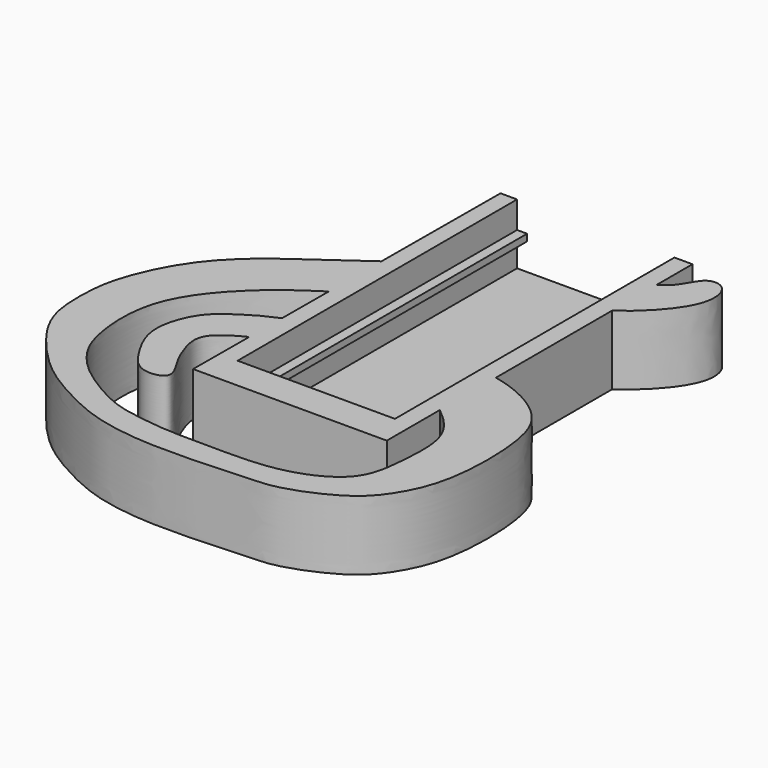
from build123d import *

# Parameters (mm, degrees)
F1_DEPTH = 50.8
F3_DEPTH = 50.8
F5_DEPTH = 44.45
F6_W     = 254.6858
F6_H     = 5
F8_DEPTH = 7.35
F7_W     = 254.6858
F7_H     = 5
F9_DEPTH = 7.35


# Not quite as in the source:
# - a feature names something its author has since deleted; it is built from what else it names


with BuildPart() as f1:
    # F0 (on Top) → F1 (new body)
    with BuildSketch(Plane.XY):
        with BuildLine():
            add(Edge.make_bspline(
                [(125.7269519745, 189.991159727), (122.3518203117, 192.7053935071), (111.2142106452, 193.3446218107), (104.5456392327, 168.8066823722), (63.3828372069, 157.6227686534), (21.7593119292, 134.7341899142), (0.3729918982, 123.8433966761), (-15.1527288368, 114.8249276639), (-32.5222819083, 102.4849064348), (-46.5725102285, 93.0684693464), (-82.8428413228, 66.746362756), (-103.7020746054, 52.59908065), (-127.8336751098, 28.9686859932), (-143.8102254505, 0.8754533738), (-152.6634719103, -25.1509877278), (-154.2263316972, -47.3151282142), (-153.2484361466, -77.7567714177), (-132.8958418183, -107.014281773), (-110.0491810359, -130.0752708141), (-88.0866600926, -143.6400857549), (-65.2385297743, -155.4769333183), (-41.5922440709, -163.1681919134), (-13.914670611, -166.3977513748), (0.1085926371, -166.5083652123), (26.8392485047, -166.7358495621), (61.2852961489, -163.9575559504), (81.9521897052, -164.4287242821), (122.6582829084, -147.5772914557), (140.1978462225, -126.7206556597), (155.9101153518, -94.4380334629), (156.0404662598, -30.3602794916), (141.7132105707, 3.4864205982), (88.6639491361, 30.0686559843), (11.8132162579, 20.380503993), (-18.3618763566, 13.3301979311), (-52.7384990739, 0.8286088804), (-69.2888621609, -9.4499896277), (-87.814391491, -22.1003193455), (-98.9611253924, -54.5390594087), (-85.3226254433, -80.4238827983), (-71.52170574, -100.1793594961), (-48.2690443764, -95.8332432139), (-57.7527638639, -80.2341547689), (-63.2820519632, -70.5245811939), (-69.3292706473, -54.6476744178), (-69.0979393699, -34.4305695104), (-2.6770546021, -7.9969048242), (42.314195006, -8.4277855233), (76.7904027335, -14.8362639415), (113.623336984, -42.8145575479), (119.3071426582, -68.2251948608), (117.588169986, -93.865138267), (114.1021059505, -125.7508497194), (80.0928160091, -144.2145120801), (45.4099166878, -147.7864485576), (16.1264360325, -146.9423859654), (-10.9926329062, -147.4579010438), (-39.004843071, -143.6649208598), (-58.6128504466, -139.0958568827), (-90.6420113734, -120.0345858112), (-105.7635321902, -103.2078654179), (-116.8591559372, -83.8529779262), (-122.0692191616, -29.7766902474), (-92.1392604492, 10.0671541536), (-65.3654050247, 33.2195527597), (-36.9417942364, 50.8675460638), (-7.1128182808, 72.0646516488), (12.800500031, 81.5981832557), (52.6243890024, 106.9180592515), (96.2625139742, 123.5069711027), (135.4755268537, 165.3473328003), (130.2770433606, 186.3320397352), (125.7269519745, 189.991159727)],
                knots=[0, 0, 0, 0, 0.0088413891, 0.0206204161, 0.0373502029, 0.0555383956, 0.0681302702, 0.0790631849, 0.090740175, 0.1017476271, 0.1188978604, 0.1323874644, 0.1471930925, 0.1620886022, 0.1755330322, 0.1877160253, 0.2017701538, 0.2171938111, 0.2320126089, 0.2451600157, 0.2582005547, 0.2713707729, 0.2848604147, 0.2945916029, 0.3079670972, 0.3231873767, 0.3352683463, 0.3520480663, 0.3655015892, 0.3808848218, 0.4014536445, 0.4167270326, 0.4360395597, 0.4587108082, 0.4735990292, 0.4888841325, 0.5003891776, 0.5123929862, 0.5269460027, 0.5408862436, 0.5532959287, 0.5634763718, 0.5728623362, 0.582057186, 0.5924855666, 0.602819313, 0.6239517883, 0.64185999, 0.6570853261, 0.6742212093, 0.687072608, 0.7002038863, 0.7143522364, 0.7298018025, 0.7452506268, 0.7592516558, 0.7728662456, 0.7864411689, 0.7982827376, 0.8139581969, 0.8262209109, 0.8382174545, 0.856822248, 0.8749632367, 0.8903214408, 0.905462531, 0.92091863, 0.9332451828, 0.9506748902, 0.969097548, 0.9880807232, 1, 1, 1, 1], degree=3))
        make_face()
    extrude(amount=F1_DEPTH)

    # F2 (on face) → F3 (join)
    with BuildSketch(Plane.XY.offset(50.8)):
        with BuildLine():
            Line((-46.8035750091, -78.4067362547), (95.1671009767, -78.409619515))
            Line((95.1671009767, -78.409619515), (95.1671009767, -29.8331879583))
            add(Edge.make_bspline(
                [(-46.5714580109, -27.2590865102), (-34.0682119102, -21.0690998309), (4.106437127, -8.0618702494), (42.314195006, -8.4277855233), (70.8109309149, -13.7247926218), (89.251013393, -25.2255814829), (95.1671009768, -29.8331879583)],
                knots=[0.611001194, 0.611001194, 0.611001194, 0.611001194, 0.6239517883, 0.64185999, 0.6570853261, 0.6655026, 0.6655026, 0.6655026, 0.6655026], degree=3))
            Line((-46.5714580109, -27.2590865102), (-46.8035750091, -78.4067362547))
        make_face()
        with BuildLine():
            add(Edge.make_bspline(
                [(-46.5714580109, -27.2590865102), (-34.0682119102, -21.0690998309), (4.106437127, -8.0618702494), (42.314195006, -8.4277855233), (70.8109309149, -13.7247926218), (89.251013393, -25.2255814829), (95.1671009768, -29.8331879583)],
                knots=[0.611001194, 0.611001194, 0.611001194, 0.611001194, 0.6239517883, 0.64185999, 0.6570853261, 0.6655026, 0.6655026, 0.6655026, 0.6655026], degree=3))
            Line((95.1671009767, -29.8331879583), (95.1671009767, 21.5398646158))
            add(Edge.make_bspline(
                [(95.1671009768, 21.5398646158), (92.8297962423, 22.0513191), (65.5031803874, 27.1489044156), (11.8132162579, 20.380503993), (-16.5897713992, 13.7442441276), (-38.2106089018, 6.0882020874), (-46.4358109558, 2.6311331304)],
                knots=[0.4338667412, 0.4338667412, 0.4338667412, 0.4338667412, 0.4360395597, 0.4587108082, 0.4735990292, 0.4857807077, 0.4857807077, 0.4857807077, 0.4857807077], degree=3))
            Line((-46.4358109558, 2.6311331304), (-46.5714580109, -27.2590865102))
        make_face()
        with BuildLine():
            add(Edge.make_bspline(
                [(95.1671009768, 21.5398646158), (92.8297962423, 22.0513191), (65.5031803874, 27.1489044156), (11.8132162579, 20.380503993), (-16.5897713992, 13.7442441276), (-38.2106089018, 6.0882020874), (-46.4358109558, 2.6311331304)],
                knots=[0.4338667412, 0.4338667412, 0.4338667412, 0.4338667412, 0.4360395597, 0.4587108082, 0.4735990292, 0.4857807077, 0.4857807077, 0.4857807077, 0.4857807077], degree=3))
            Line((95.1671009767, 21.5398646158), (95.1671009767, 127.8310488696))
            add(Edge.make_bspline(
                [(-46.2426435255, 45.1961333015), (-43.0776503309, 47.2670156911), (-29.9013887118, 55.8706081698), (-7.1128182808, 72.0646516488), (12.800500031, 81.5981832557), (52.4019975541, 106.7766636209), (80.7274218698, 117.6009223881), (95.1671009766, 127.8310488696)],
                knots=[0.9004525479, 0.9004525479, 0.9004525479, 0.9004525479, 0.905462531, 0.92091863, 0.9332451828, 0.9506748902, 0.968828499, 0.968828499, 0.968828499, 0.968828499], degree=3))
            Line((-46.2426435254, 45.1961333015), (-46.4358109558, 2.6311331304))
        make_face()
        with BuildLine():
            Line((-45.5328990233, 201.590380485), (-46.0245758076, 93.2479835951))
            add(Edge.make_bspline(
                [(95.1671009766, 168.8222056765), (86.9990973718, 163.9239706682), (59.8217062278, 155.6645196519), (21.7593119292, 134.7341899142), (0.3729918982, 123.8433966761), (-15.1527288368, 114.8249276639), (-32.3304338629, 102.6212029153), (-40.2604651432, 97.2989166807), (-46.0245758077, 93.2479835951)],
                knots=[0.0246851562, 0.0246851562, 0.0246851562, 0.0246851562, 0.0373502029, 0.0555383956, 0.0681302702, 0.0790631849, 0.090740175, 0.1013763208, 0.1013763208, 0.1013763208, 0.1013763208], degree=3))
            Line((95.1671009767, 168.8222056765), (95.1671009767, 201.590380485))
            Line((95.1671009767, 201.590380485), (-45.5328990233, 201.590380485))
        make_face()
    extrude(amount=-F3_DEPTH)

    # F4 (on face) → F5 (cut)
    with BuildSketch(Plane.XY.offset(50.8)):
        with BuildLine():
            Line((81.9325018531, 162.6230259561), (81.9321837852, 201.590380485))
            Line((81.9321837852, 201.590380485), (-33.3657265927, 201.590380485))
            Line((-33.3657265927, 201.590380485), (-33.3657265927, 101.998818935))
            add(Edge.make_bspline(
                [(81.9325018532, 162.6230259561), (76.4815710378, 160.4783865935), (54.5886080956, 152.7868638586), (21.7593119292, 134.7341899142), (0.3729918982, 123.8433966761), (-15.1527288368, 114.8249276639), (-27.4360360639, 106.098377745), (-32.8786985755, 102.3348578929), (-33.3657265927, 101.998818935)],
                knots=[0.0306583102, 0.0306583102, 0.0306583102, 0.0306583102, 0.0373502029, 0.0555383956, 0.0681302702, 0.0790631849, 0.090740175, 0.091903612, 0.091903612, 0.091903612, 0.091903612], degree=3))
        make_face()
        with BuildLine():
            Line((81.9328531355, 119.5864658858), (81.9325018531, 162.6230259561))
            add(Edge.make_bspline(
                [(81.9325018532, 162.6230259561), (76.4815710378, 160.4783865935), (54.5886080956, 152.7868638586), (21.7593119292, 134.7341899142), (0.3729918982, 123.8433966761), (-15.1527288368, 114.8249276639), (-27.4360360639, 106.098377745), (-32.8786985755, 102.3348578929), (-33.3657265927, 101.998818935)],
                knots=[0.0306583102, 0.0306583102, 0.0306583102, 0.0306583102, 0.0373502029, 0.0555383956, 0.0681302702, 0.0790631849, 0.090740175, 0.091903612, 0.091903612, 0.091903612, 0.091903612], degree=3))
            Line((-33.3657265927, 101.998818935), (-33.3657265927, 53.7188803265))
            add(Edge.make_bspline(
                [(-33.3657265927, 53.7188803265), (-24.1976873803, 59.9141802901), (-6.4010596607, 72.405407177), (12.800500031, 81.5981832557), (47.8214872557, 103.8643927265), (71.8786453995, 114.0385140692), (81.9328531356, 119.5864658858)],
                knots=[0.9070785493, 0.9070785493, 0.9070785493, 0.9070785493, 0.92091863, 0.9332451828, 0.9506748902, 0.9632870003, 0.9632870003, 0.9632870003, 0.9632870003], degree=3))
        make_face()
        with BuildLine():
            Line((81.9336362003, 23.6510812759), (81.9328531355, 119.5864658858))
            add(Edge.make_bspline(
                [(-33.3657265927, 53.7188803265), (-24.1976873803, 59.9141802901), (-6.4010596607, 72.405407177), (12.800500031, 81.5981832557), (47.8214872557, 103.8643927265), (71.8786453995, 114.0385140692), (81.9328531356, 119.5864658858)],
                knots=[0.9070785493, 0.9070785493, 0.9070785493, 0.9070785493, 0.92091863, 0.9332451828, 0.9506748902, 0.9632870003, 0.9632870003, 0.9632870003, 0.9632870003], degree=3))
            Line((-33.3657265927, 53.7188803265), (-33.3657265927, 7.6883592702))
            add(Edge.make_bspline(
                [(81.9336362003, 23.6510812759), (57.830614396, 26.1765022465), (10.7986173979, 20.1434464772), (-13.125120387, 14.5537478579), (-28.8279560716, 9.3170993456), (-33.3657265927, 7.6883592702)],
                knots=[0.4378163908, 0.4378163908, 0.4378163908, 0.4378163908, 0.4587108082, 0.4735990292, 0.4797131869, 0.4797131869, 0.4797131869, 0.4797131869], degree=3))
        make_face()
        with BuildLine():
            Line((81.9340007063, -21.0055399792), (81.9336362003, 23.6510812759))
            add(Edge.make_bspline(
                [(81.9336362003, 23.6510812759), (57.830614396, 26.1765022465), (10.7986173979, 20.1434464772), (-13.125120387, 14.5537478579), (-28.8279560716, 9.3170993456), (-33.3657265927, 7.6883592702)],
                knots=[0.4378163908, 0.4378163908, 0.4378163908, 0.4378163908, 0.4587108082, 0.4735990292, 0.4797131869, 0.4797131869, 0.4797131869, 0.4797131869], degree=3))
            Line((-33.3657265927, 7.6883592702), (-33.3657265927, -21.4725641799))
            add(Edge.make_bspline(
                [(-33.3657265928, -21.4725641798), (-23.8189305052, -17.7459515172), (7.6205617994, -8.0955249824), (42.314195006, -8.4277855233), (66.7171883615, -12.9638428964), (80.0817272052, -19.9593320041), (81.9340007063, -21.0055399792)],
                knots=[0.6152397413, 0.6152397413, 0.6152397413, 0.6152397413, 0.6239517883, 0.64185999, 0.6570853261, 0.6595335541, 0.6595335541, 0.6595335541, 0.6595335541], degree=3))
        make_face()
        with BuildLine():
            Line((81.9342733835, -54.4119611247), (81.9340007063, -21.0055399792))
            add(Edge.make_bspline(
                [(-33.3657265928, -21.4725641798), (-23.8189305052, -17.7459515172), (7.6205617994, -8.0955249824), (42.314195006, -8.4277855233), (66.7171883615, -12.9638428964), (80.0817272052, -19.9593320041), (81.9340007063, -21.0055399792)],
                knots=[0.6152397413, 0.6152397413, 0.6152397413, 0.6152397413, 0.6239517883, 0.64185999, 0.6570853261, 0.6595335541, 0.6595335541, 0.6595335541, 0.6595335541], degree=3))
            Line((-33.3657265927, -21.4725641799), (-33.3657265927, -54.409619515))
            Line((-33.3657265927, -54.409619515), (81.9342733835, -54.4119611247))
        make_face()
    extrude(amount=-F5_DEPTH, mode=Mode.SUBTRACT)

    # F6 (on face) → F8 (join)
    with BuildSketch(Plane.YZ.offset(-33.3657265927)):
        with Locations((74.247480485, 28.575)):
            Rectangle(F6_W, F6_H)
    extrude(amount=F8_DEPTH)

    # F7 (on face) → F9 (join)
    with BuildSketch(Plane(origin=(81.9338292449, 0.0006687782, 0), x_dir=(8.1624e-06, -1, 0), z_dir=(-1, -8.1624e-06, 0))):
        with Locations((-74.2468117135, 28.575)):
            Rectangle(F7_W, F7_H)
    extrude(amount=F9_DEPTH)


solid = f1.part
